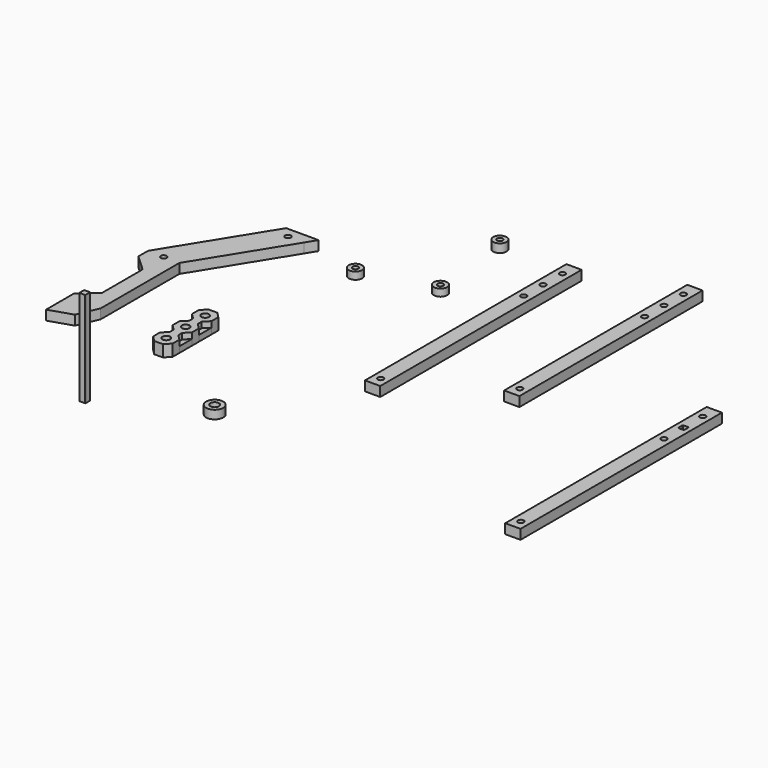
from build123d import *

# Parameters (mm, degrees)
F1_DEPTH  = 5.08
F0_W      = 8
F0_H      = 117
F0_H_2    = 15
F0_R      = 1.5
F0_H_3    = 105
F0_W_2    = 3.15
F0_H_4    = 3.15
F2_DEPTH  = 50
F0_R_2    = 3.5
F3_DEPTH  = 4.45
F0_R_3    = 4.5
F0_R_4    = 2.25
F4_R      = 0.25
F5_R      = 3.5
F5_R_2    = 1.5
F6_DEPTH  = 3.815
F8_DEPTH  = 3.1
F7_W      = 2.25
F7_H      = 2.55
F9_DEPTH  = 6.15
F10_DEPTH = 3.764


# Not quite as in the source:
# - a feature names something its author has since deleted; it is built from what else it names


with BuildPart() as f1:
    # F0 (on Top) → F1 (new body)
    with BuildSketch(Plane.XY):
        with BuildLine():
            Line((-50.949690631, 43.8997100926), (-67.949690631, 43.8997100926))
            Line((-67.949690631, 43.8997100926), (-71.2368406563, 38.5939453388))
            Line((-71.2368406563, 38.5939453388), (-64.2368406563, 38.5939453388))
            ThreePointArc((-64.2368406563, 38.5939453388), (-62.7368406563, 40.0939453388), (-61.2368406563, 38.5939453388))
            Line((-61.2368406563, 38.5939453388), (-54.2368406563, 38.5939453388))
            Line((-54.2368406563, 38.5939453388), (-50.949690631, 43.8997100926))
        make_face()
        Polygon((-90.9492363239, -13.4048849161), (-99.5492363239, -13.4048849161), (-90.9492363239, -21.4048934984), align=None)
        Polygon((-90.9492363239, -55.9028989029), (-90.9492363239, -47.8827440429), (-99.5708935492, -55.9028989029), align=None)
        with BuildLine():
            Line((-64.2368406563, 38.5939453388), (-71.2368406563, 38.5939453388))
            Line((-71.2368406563, 38.5939453388), (-99.5492363239, -7.1048849161))
            Line((-99.5492363239, -7.1048849161), (-92.680417628, -7.2793228948))
            ThreePointArc((-92.680417628, -7.2793228948), (-91.1618589797, -5.8175249342), (-89.6809010977, -7.3174040619))
            ThreePointArc((-89.6809010977, -7.3174040619), (-89.6810219699, -7.3364461799), (-89.6813845673, -7.3554852291))
            Line((-89.6813845673, -7.3554852291), (-82.8125658714, -7.5299232078))
            Line((-82.8125658714, -7.5299232078), (-54.2368406563, 38.5939453388))
            Line((-54.2368406563, 38.5939453388), (-61.2368406563, 38.5939453388))
            ThreePointArc((-61.2368406563, 38.5939453388), (-62.7368406563, 37.0939453388), (-64.2368406563, 38.5939453388))
        make_face()
        with BuildLine():
            Line((-92.680417628, -7.2793228948), (-99.5492363239, -7.1048849161))
            Line((-99.5492363239, -7.1048849161), (-99.5492363239, -13.4048849161))
            Line((-99.5492363239, -13.4048849161), (-90.9492363239, -13.4048849161))
            Line((-90.9492363239, -13.4048849161), (-90.9492363239, -21.4048934984))
            Line((-90.9492363239, -21.4048934984), (-90.9492363239, -47.8827440429))
            Line((-90.9492363239, -47.8827440429), (-90.9492363239, -55.9028989029))
            Line((-90.9492363239, -55.9028989029), (-99.5708935492, -55.9028989029))
            Line((-99.5708935492, -55.9028989029), (-99.5708935492, -73.9028989029))
            Line((-99.5708935492, -73.9028989029), (-87.5764183456, -70.0438103329))
            Line((-87.5764183456, -70.0438103329), (-82.8125658714, -59.0299232078))
            Line((-82.8125658714, -59.0299232078), (-82.8125658714, -7.5299232078))
            Line((-82.8125658714, -7.5299232078), (-89.6813845673, -7.3554852291))
            ThreePointArc((-89.6813845673, -7.3554852291), (-91.2189822648, -8.8169205923), (-92.680417628, -7.2793228948))
        make_face()
    extrude(amount=F1_DEPTH)


with BuildPart() as f1b:
    # F0 (on Top) → F1, piece 2 (new body)
    with BuildSketch(Plane.XY):
        with Locations((45.5790795386, 17.1512553096)):
            Rectangle(F0_W, F0_H)
        with BuildLine():
            ThreePointArc((47.0790795386, -36.0787446904), (44.5184193668, -37.1394048622), (45.5790795386, -34.5787446904))
            ThreePointArc((45.5790795386, -34.5787446904), (46.6397397104, -35.0180845186), (47.0790795386, -36.0787446904))
        make_face(mode=Mode.SUBTRACT)
        with BuildLine():
            ThreePointArc((45.5790795386, 56.1812553096), (44.0790795386, 57.6812553096), (45.5790795386, 59.1812553096))
            ThreePointArc((45.5790795386, 59.1812553096), (46.6397397104, 58.7419154814), (47.0790795386, 57.6812553096))
            ThreePointArc((47.0790795386, 57.6812553096), (46.6397397104, 56.6205951378), (45.5790795386, 56.1812553096))
        make_face(mode=Mode.SUBTRACT)
        with BuildLine():
            ThreePointArc((47.0790795386, 70.3812553096), (46.6397397104, 69.3205951378), (45.5790795386, 68.8812553096))
            ThreePointArc((45.5790795386, 68.8812553096), (44.5184193668, 71.4419154814), (47.0790795386, 70.3812553096))
        make_face(mode=Mode.SUBTRACT)
        with Locations((45.5790795386, 83.1512553096)):
            Rectangle(F0_W, F0_H_2)
        with Locations((45.5790795386, 83.0812553096)):
            Circle(F0_R, mode=Mode.SUBTRACT)
    extrude(amount=F1_DEPTH)


with BuildPart() as f1c:
    # F0 (on Top) → F1, piece 3 (new body)
    with BuildSketch(Plane.XY):
        with Locations((95.6552401185, 39.7728151456)):
            Rectangle(F0_W, F0_H_3)
        with BuildLine():
            ThreePointArc((97.1552401185, -7.4771848544), (94.5945799467, -8.5378450262), (95.6552401185, -5.9771848544))
            ThreePointArc((95.6552401185, -5.9771848544), (96.7159002903, -6.4165246827), (97.1552401185, -7.4771848544))
        make_face(mode=Mode.SUBTRACT)
        with BuildLine():
            ThreePointArc((95.6552401185, 72.8228151456), (94.1552401185, 74.3228151456), (95.6552401185, 75.8228151456))
            ThreePointArc((95.6552401185, 75.8228151456), (96.7159002903, 75.3834753173), (97.1552401185, 74.3228151456))
            ThreePointArc((97.1552401185, 74.3228151456), (96.7159002903, 73.2621549738), (95.6552401185, 72.8228151456))
        make_face(mode=Mode.SUBTRACT)
        with BuildLine():
            ThreePointArc((97.1552401185, 87.0228151456), (96.7159002903, 85.9621549738), (95.6552401185, 85.5228151456))
            ThreePointArc((95.6552401185, 85.5228151456), (94.5945799467, 88.0834753173), (97.1552401185, 87.0228151456))
        make_face(mode=Mode.SUBTRACT)
        with Locations((95.6552401185, 99.7728151456)):
            Rectangle(F0_W, F0_H_2)
        with Locations((95.6552401185, 99.7228151456)):
            Circle(F0_R, mode=Mode.SUBTRACT)
    extrude(amount=F1_DEPTH)


with BuildPart() as f1d:
    # F0 (on Top) → F1, piece 4 (new body)
    with BuildSketch(Plane.XY):
        with Locations((169.5275753736, -45.8602230102)):
            Rectangle(F0_W, F0_H)
        with BuildLine():
            ThreePointArc((171.0275753736, -99.1102230102), (168.4669152019, -100.170883182), (169.5275753736, -97.6102230102))
            ThreePointArc((169.5275753736, -97.6102230102), (170.5882355454, -98.0495628384), (171.0275753736, -99.1102230102))
        make_face(mode=Mode.SUBTRACT)
        with BuildLine():
            ThreePointArc((171.0275753736, -5.3102230102), (170.5882355454, -6.370883182), (169.5275753736, -6.8102230102))
            ThreePointArc((169.5275753736, -6.8102230102), (168.0275753736, -5.3102230102), (169.5275753736, -3.8102230102))
            ThreePointArc((169.5275753736, -3.8102230102), (170.5882355454, -4.2495628384), (171.0275753736, -5.3102230102))
        make_face(mode=Mode.SUBTRACT)
        with BuildLine():
            ThreePointArc((170.8877224245, 5.7897769898), (170.252144211, 5.4187366554), (169.5275753736, 5.2897769898))
            ThreePointArc((169.5275753736, 5.2897769898), (168.8030065363, 5.4187366554), (168.1674283228, 5.7897769898))
            Line((168.1674283228, 5.7897769898), (167.9275753736, 5.7897769898))
            Line((167.9275753736, 5.7897769898), (167.9275753736, 6.0296299389))
            ThreePointArc((167.9275753736, 6.0296299389), (167.4275753736, 7.3897769898), (167.9275753736, 8.7499240407))
            Line((167.9275753736, 8.7499240407), (167.9275753736, 8.9897769898))
            Line((167.9275753736, 8.9897769898), (168.1674283228, 8.9897769898))
            ThreePointArc((168.1674283228, 8.9897769898), (169.5275753736, 9.4897769898), (170.8877224245, 8.9897769898))
            Line((170.8877224245, 8.9897769898), (171.1275753736, 8.9897769898))
            Line((171.1275753736, 8.9897769898), (171.1275753736, 8.7499240407))
            ThreePointArc((171.1275753736, 8.7499240407), (171.4986157081, 8.1143458271), (171.6275753736, 7.3897769898))
            ThreePointArc((171.6275753736, 7.3897769898), (171.4986157081, 6.6652081525), (171.1275753736, 6.0296299389))
            Line((171.1275753736, 6.0296299389), (171.1275753736, 5.7897769898))
            Line((171.1275753736, 5.7897769898), (170.8877224245, 5.7897769898))
        make_face(mode=Mode.SUBTRACT)
        with Locations((169.5275753736, 20.1397769898)):
            Rectangle(F0_W, F0_H_2)
        with Locations((169.5275753736, 20.0897769898)):
            Circle(F0_R, mode=Mode.SUBTRACT)
        with BuildLine():
            ThreePointArc((170.8877224245, 8.9897769898), (169.5275753736, 9.4897769898), (168.1674283228, 8.9897769898))
            Line((168.1674283228, 8.9897769898), (170.8877224245, 8.9897769898))
        make_face()
        with BuildLine():
            ThreePointArc((167.9275753736, 8.7499240407), (167.4275753736, 7.3897769898), (167.9275753736, 6.0296299389))
            Line((167.9275753736, 6.0296299389), (167.9275753736, 8.7499240407))
        make_face()
        with BuildLine():
            Line((171.1275753736, 8.7499240407), (171.1275753736, 6.0296299389))
            ThreePointArc((171.1275753736, 6.0296299389), (171.4986157081, 6.6652081525), (171.6275753736, 7.3897769898))
            ThreePointArc((171.6275753736, 7.3897769898), (171.4986157081, 8.1143458271), (171.1275753736, 8.7499240407))
        make_face()
        with BuildLine():
            Line((169.5275753736, 5.7897769898), (169.5275753736, 5.2897769898))
            ThreePointArc((169.5275753736, 5.2897769898), (170.252144211, 5.4187366554), (170.8877224245, 5.7897769898))
            Line((170.8877224245, 5.7897769898), (169.5275753736, 5.7897769898))
        make_face()
        with BuildLine():
            ThreePointArc((168.1674283228, 5.7897769898), (168.8030065363, 5.4187366554), (169.5275753736, 5.2897769898))
            Line((169.5275753736, 5.2897769898), (169.5275753736, 5.7897769898))
            Line((169.5275753736, 5.7897769898), (168.1674283228, 5.7897769898))
        make_face()
        with BuildLine():
            ThreePointArc((170.8877224245, 8.9897769898), (171.0124996141, 8.8747012303), (171.1275753736, 8.7499240407))
            Line((171.1275753736, 8.7499240407), (171.1275753736, 8.9897769898))
            Line((171.1275753736, 8.9897769898), (170.8877224245, 8.9897769898))
        make_face()
        with BuildLine():
            Line((167.9275753736, 8.9897769898), (167.9275753736, 8.7499240407))
            ThreePointArc((167.9275753736, 8.7499240407), (168.0426511332, 8.8747012303), (168.1674283228, 8.9897769898))
            Line((168.1674283228, 8.9897769898), (167.9275753736, 8.9897769898))
        make_face()
        with BuildLine():
            Line((167.9275753736, 5.7897769898), (168.1674283228, 5.7897769898))
            ThreePointArc((168.1674283228, 5.7897769898), (168.0426511332, 5.9048527493), (167.9275753736, 6.0296299389))
            Line((167.9275753736, 6.0296299389), (167.9275753736, 5.7897769898))
        make_face()
        with BuildLine():
            ThreePointArc((171.1275753736, 6.0296299389), (171.0124996141, 5.9048527493), (170.8877224245, 5.7897769898))
            Line((170.8877224245, 5.7897769898), (171.1275753736, 5.7897769898))
            Line((171.1275753736, 5.7897769898), (171.1275753736, 6.0296299389))
        make_face()
    extrude(amount=F1_DEPTH)


with BuildPart() as f2:
    # F0 (on Top) → F2 (new body)
    with BuildSketch(Plane.XY):
        with Locations((-42.7516108632, -119.568117547)):
            Rectangle(F0_W_2, F0_H_4)
        with Locations((-42.7516108632, -119.568117547)):
            Circle(F0_R, mode=Mode.SUBTRACT)
        with Locations((-42.7516108632, -119.568117547)):
            Circle(F0_R)
    extrude(amount=F2_DEPTH)

    # F4
    f4_edges = [f2.edges().sort_by_distance(p)[0] for p in [
        (-41.176611, -121.143118, 25),
        (-44.326611, -117.993118, 25),
        (-44.326611, -121.143118, 25),
        (-41.176611, -117.993118, 25),
    ]]
    fillet(f4_edges, radius=F4_R)


with BuildPart() as f3:
    # F0 (on Top) → F3 (new body)
    with BuildSketch(Plane.XY):
        with Locations((5.9054424055, 91.6430652142)):
            Circle(F0_R_2)
        with Locations((5.9054424055, 91.6430652142)):
            Circle(F0_R, mode=Mode.SUBTRACT)
    extrude(amount=F3_DEPTH)


with BuildPart() as f3b:
    # F0 (on Top) → F3, piece 2 (new body)
    with BuildSketch(Plane.XY):
        with Locations((6.2566562556, -95.6798642874)):
            Circle(F0_R_3)
        with Locations((6.2566562556, -95.6798642874)):
            Circle(F0_R_4, mode=Mode.SUBTRACT)
    extrude(amount=F3_DEPTH)


with BuildPart() as f6:
    # F5 (on Top) → F6 (new body)
    with BuildSketch(Plane.XY):
        with Locations((-25.4324208945, 36.1619368196)):
            Circle(F5_R)
        with Locations((-25.4324208945, 36.1619368196)):
            Circle(F5_R_2, mode=Mode.SUBTRACT)
    extrude(amount=F6_DEPTH)


with BuildPart() as f8:
    # F7 (on Top) → F8 (new body)
    with BuildSketch(Plane.XY):
        Polygon((-39.0240414023, -49.4567692398), (-39.0240414023, -41.1911208631), (-41.8740414023, -44.0489450514), (-41.8740414023, -46.5989450514), align=None)
    extrude(amount=F8_DEPTH)


with BuildPart() as f8b:
    # F7 (on Top) → F8, piece 2 (new body)
    with BuildSketch(Plane.XY):
        Polygon((-46.3740414023, -46.5989450514), (-46.3740414023, -44.0489450514), (-49.2240414023, -41.1911208631), (-49.2240414023, -49.4567692398), align=None)
    extrude(amount=F8_DEPTH)


with BuildPart() as f8c:
    # F7 (on Top) → F8, piece 3 (new body)
    with BuildSketch(Plane.XY):
        Polygon((-46.3740414023, -56.7989450514), (-49.2240414023, -53.9567692398), (-49.2240414023, -62.1911208631), (-46.3740414023, -59.3489450514), align=None)
    extrude(amount=F8_DEPTH)


with BuildPart() as f8d:
    # F7 (on Top) → F8, piece 4 (new body)
    with BuildSketch(Plane.XY):
        Polygon((-39.0240414023, -62.1911208631), (-39.0240414023, -53.9567692398), (-41.8740414023, -56.7989450514), (-41.8740414023, -59.3489450514), align=None)
    extrude(amount=F8_DEPTH)


with BuildPart() as f9:
    # F7 (on Top) → F9 (new body)
    with BuildSketch(Plane.XY):
        with BuildLine():
            ThreePointArc((-44.1240414023, -40.9489450514), (-45.5382549647, -37.5347314891), (-42.1240414023, -38.9489450514))
            Line((-42.1240414023, -38.9489450514), (-39.0240414023, -38.9489450514))
            Line((-39.0240414023, -38.9489450514), (-39.0240414023, -36.6911208631))
            Line((-39.0240414023, -36.6911208631), (-41.8740414023, -33.8489450514))
            Line((-41.8740414023, -33.8489450514), (-46.3740414023, -33.8489450514))
            Line((-46.3740414023, -33.8489450514), (-49.2240414023, -36.6911208631))
            Line((-49.2240414023, -36.6911208631), (-49.2240414023, -41.1911208631))
            Line((-49.2240414023, -41.1911208631), (-46.3740414023, -44.0489450514))
            Line((-46.3740414023, -44.0489450514), (-44.1240414023, -44.0489450514))
            Line((-44.1240414023, -44.0489450514), (-44.1240414023, -40.9489450514))
        make_face()
        with BuildLine():
            Line((-39.0240414023, -38.9489450514), (-42.1240414023, -38.9489450514))
            ThreePointArc((-42.1240414023, -38.9489450514), (-42.70982784, -40.3631586138), (-44.1240414023, -40.9489450514))
            Line((-44.1240414023, -40.9489450514), (-44.1240414023, -44.0489450514))
            Line((-44.1240414023, -44.0489450514), (-41.8740414023, -44.0489450514))
            Line((-41.8740414023, -44.0489450514), (-39.0240414023, -41.1911208631))
            Line((-39.0240414023, -41.1911208631), (-39.0240414023, -38.9489450514))
        make_face()
        with BuildLine():
            Line((-41.8740414023, -46.5989450514), (-44.1240414023, -46.5989450514))
            Line((-44.1240414023, -46.5989450514), (-44.1240414023, -49.6989450514))
            ThreePointArc((-44.1240414023, -49.6989450514), (-42.70982784, -50.2847314891), (-42.1240414023, -51.6989450514))
            ThreePointArc((-42.1240414023, -51.6989450514), (-42.70982784, -53.1131586138), (-44.1240414023, -53.6989450514))
            Line((-44.1240414023, -53.6989450514), (-44.1240414023, -56.7989450514))
            Line((-44.1240414023, -56.7989450514), (-41.8740414023, -56.7989450514))
            Line((-41.8740414023, -56.7989450514), (-39.0240414023, -53.9567692398))
            Line((-39.0240414023, -53.9567692398), (-39.0240414023, -49.4567692398))
            Line((-39.0240414023, -49.4567692398), (-41.8740414023, -46.5989450514))
        make_face()
        with BuildLine():
            Line((-44.1240414023, -49.6989450514), (-44.1240414023, -46.5989450514))
            Line((-44.1240414023, -46.5989450514), (-46.3740414023, -46.5989450514))
            Line((-46.3740414023, -46.5989450514), (-49.2240414023, -49.4567692398))
            Line((-49.2240414023, -49.4567692398), (-49.2240414023, -53.9567692398))
            Line((-49.2240414023, -53.9567692398), (-46.3740414023, -56.7989450514))
            Line((-46.3740414023, -56.7989450514), (-44.1240414023, -56.7989450514))
            Line((-44.1240414023, -56.7989450514), (-44.1240414023, -53.6989450514))
            ThreePointArc((-44.1240414023, -53.6989450514), (-46.1240414023, -51.6989450514), (-44.1240414023, -49.6989450514))
        make_face()
        Polygon((-39.0240414023, -66.6911208631), (-39.0240414023, -62.1911208631), (-41.8740414023, -59.3489450514), (-44.1240414023, -59.3489450514), (-46.3740414023, -59.3489450514), (-49.2240414023, -62.1911208631), (-49.2240414023, -66.6911208631), (-46.3740414023, -69.5489450514), (-41.8740414023, -69.5489450514), align=None)
        with BuildLine():
            ThreePointArc((-42.1240414023, -64.4489450514), (-45.5382549647, -65.8631586138), (-44.1240414023, -62.4489450514))
            ThreePointArc((-44.1240414023, -62.4489450514), (-42.70982784, -63.0347314891), (-42.1240414023, -64.4489450514))
        make_face(mode=Mode.SUBTRACT)
        with Locations((-45.2490414023, -45.3239450514)):
            Rectangle(F7_W, F7_H)
        with Locations((-42.9990414023, -45.3239450514)):
            Rectangle(F7_W, F7_H)
        with Locations((-45.2490414023, -58.0739450514)):
            Rectangle(F7_W, F7_H)
        with Locations((-42.9990414023, -58.0739450514)):
            Rectangle(F7_W, F7_H)
    extrude(amount=F9_DEPTH)


with BuildPart() as f10:
    # F5 (on Top) → F10 (new body)
    with BuildSketch(Plane.XY):
        with Locations((11.1080519855, 46.2102368474)):
            Circle(F5_R)
        with Locations((11.1080519855, 46.2102368474)):
            Circle(F5_R_2, mode=Mode.SUBTRACT)
    extrude(amount=F10_DEPTH)


solid = Compound([f1.part, f1b.part, f1c.part, f1d.part, f2.part, f3.part, f3b.part, f6.part, f8.part, f8b.part, f8c.part, f8d.part, f9.part, f10.part])
